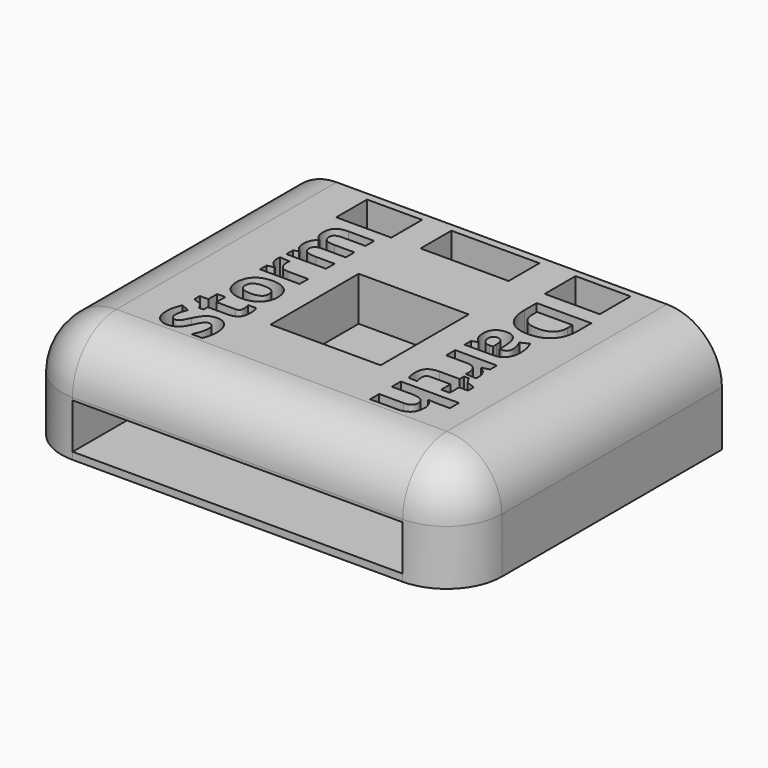
from build123d import *

# Parameters (mm, degrees)
F0_W         = 101.6
F0_H         = 76.2
F1_DEPTH     = 25.4
F2_R         = 12.7
F3_W         = 25.4
F3_H         = 25.4
F4_DEPTH     = 10.16
F6_TEXT_SIZE = 16.7648120456
F5_TEXT_SIZE = 17.6427176036
F7_DEPTH     = 12.7
F8_W         = 76.0942026973
F8_H         = 10.4400189593
F9_DEPTH     = 25.4
F10_W        = 12.7
F10_H        = 8.89
F11_DEPTH    = 20.32
F12_W        = 20.32
F12_H        = 8.89
F13_W        = 12.7
F13_H        = 8.89
F14_DEPTH    = 20.32


# Not quite as in the source:
# - Text() gives the source's letters only with a copy of the font that has no kerning and outlines rounded to 1/6400 em; it was checked with that copy


with BuildPart() as f1:
    # F0 (on Top) → F1 (new body)
    with BuildSketch(Plane.XY):
        Rectangle(F0_W, F0_H)
    extrude(amount=F1_DEPTH)

    # F2
    f2_edges = [f1.edges().sort_by_distance(p)[0] for p in [
        (-50.8, -38.1, 12.7),
        (0, -38.1, 25.4),
        (50.8, -38.1, 12.7),
        (50.8, 0, 25.4),
        (-50.8, 0, 25.4),
    ]]
    fillet(f2_edges, radius=F2_R)

    # F3 (on face) → F4 (cut)
    with BuildSketch(Plane.XY.offset(25.4)):
        Rectangle(F3_W, F3_H)
    extrude(amount=-F4_DEPTH, mode=Mode.SUBTRACT)

    # F6 (on face) + F5 (on face) → F7 (cut)
    with BuildSketch(Plane.XY.offset(25.4)):
        with Locations(Location((-18.5153097821, -25.2607837319), (0, 0, 90))):
            Text('Storm', F6_TEXT_SIZE, font='Open Sans', font_style=FontStyle.BOLD, text_align=(TextAlign.LEFT, TextAlign.BOTTOM))
    with BuildSketch(Plane.XY.offset(25.4)):
        with Locations(Location((19.4967825695, 25.400000307), (0, 0, -90))):
            Text('Darth', F5_TEXT_SIZE, font='Open Sans', font_style=FontStyle.BOLD, text_align=(TextAlign.LEFT, TextAlign.BOTTOM))
    extrude(amount=-F7_DEPTH, mode=Mode.SUBTRACT)

    # F8 (on face) → F9 (cut)
    with BuildSketch(Plane.XZ.offset(38.1)):
        with Locations((0, 6.8688592874)):
            Rectangle(F8_W, F8_H)
    extrude(amount=-F9_DEPTH, mode=Mode.SUBTRACT)

    # F10 (on face) → F11 (cut)
    with BuildSketch(Plane.XY.offset(25.4)):
        with Locations((-23.2667587585, 31.8235255849)):
            Rectangle(F10_W, F10_H)
    extrude(amount=-F11_DEPTH, mode=Mode.SUBTRACT)

    # F12 (on face) + F13 (on face) → F14 (cut)
    with BuildSketch(Plane.XY.offset(25.4)):
        with Locations((0, 31.8235255849)):
            Rectangle(F12_W, F12_H)
    with BuildSketch(Plane.XY.offset(25.4)):
        with Locations((24.7321538627, 31.9622501819)):
            Rectangle(F13_W, F13_H)
    extrude(amount=-F14_DEPTH, mode=Mode.SUBTRACT)


solid = f1.part
